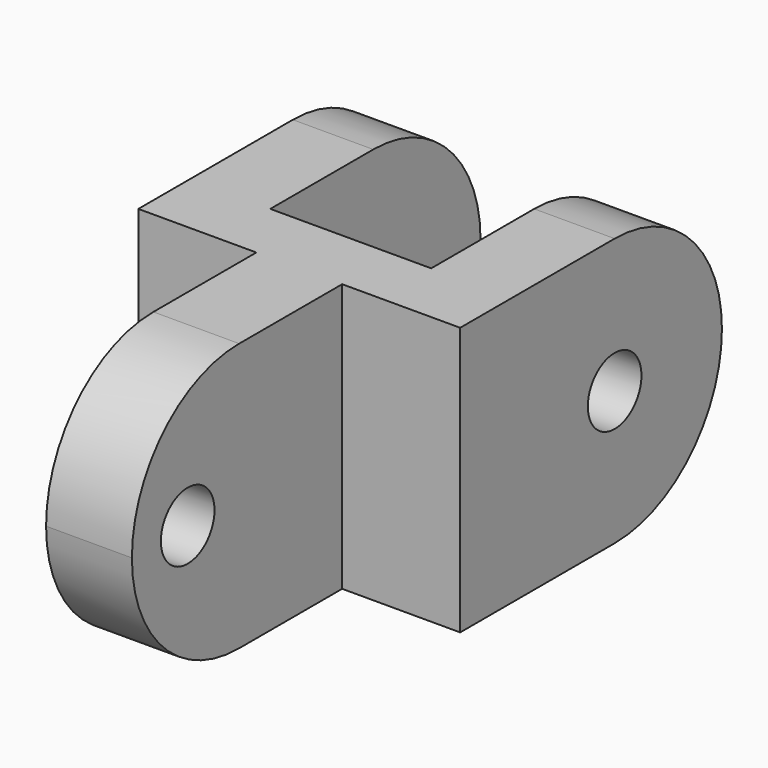
from build123d import *

# Parameters (mm, degrees)
F1_DEPTH = 1270
F2_R     = 634.99999
F4_D     = 317.5
F6_D     = 317.5


# Not quite as in the source:
# - a fillet or chamfer is up to 0.001 mm smaller than in the source, because OpenCascade refuses the exact size


with BuildPart() as f1:
    # F0 (on Top) → F1 (new body)
    with BuildSketch(Plane.XY):
        Polygon((381, 0), (0, 0), (0, -1549.4), (558.8, -1549.4), (558.8, -2794), (965.2, -2794), (965.2, -1549.4), (1524, -1549.4), (1524, 0), (1143, 0), (1143, -1244.6), (381, -1244.6), align=None)
    extrude(amount=F1_DEPTH)

    # F2 (radius 635 in the source; OpenCascade refuses exactly that, so slightly less here)
    f2_edges = [f1.edges().sort_by_distance(p)[0] for p in [
        (190.5, 0, 1270),
        (190.5, 0, 0),
        (1333.5, 0, 1270),
        (1333.5, 0, 0),
        (762, -2794, 1270),
        (762, -2794, 0),
    ]]
    fillet(f2_edges, radius=F2_R)

    # F4 (through all)
    with Locations(Plane(origin=(558.8, 0, 0), x_dir=(0, -1, 0), z_dir=(-1, 0, 0))):
        with Locations((2463.8, 635)):
            Hole(F4_D / 2)

    # F6 (through all)
    with Locations(Plane.YZ.offset(1524)):
        with Locations((-635, 635)):
            Hole(F6_D / 2)


solid = f1.part
